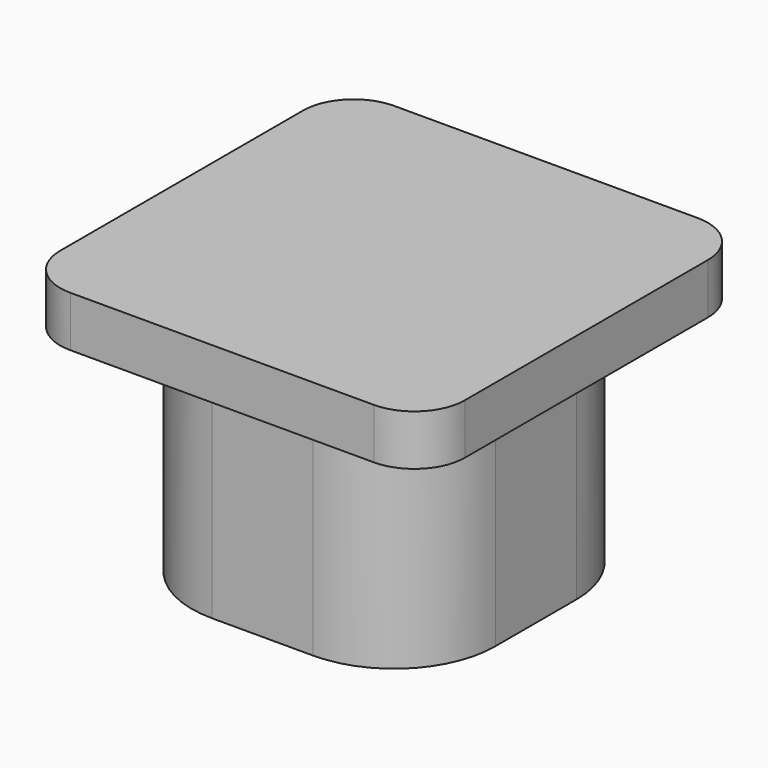
from build123d import *

# Parameters (mm, degrees)
F1_DEPTH     = 56.134
F3_DEPTH     = 12.7
F4_T         = 6.35
F4_T3_DEPTH  = 38.1
F4_T5_DEPTH  = 38.1
F4_T8_ANGLE  = 90.000000001
F4_T10_ANGLE = 90.000000001
F4_T12_ANGLE = 90.000000001
F4_T14_ANGLE = 90.000000001


# Not quite as in the source:
# - a shell that OpenCascade refuses in one call is made with other operations: the cavity is built on its own and cut out


with BuildPart() as f1:
    # F0 (on Top) → F1 (new body)
    with BuildSketch(Plane.XY):
        with BuildLine():
            ThreePointArc((-38.1, -12.7), (-30.6605122421, -30.6605122421), (-12.7, -38.1))
            Line((-12.7, -38.1), (12.7, -38.1))
            ThreePointArc((12.7, -38.1), (30.6605122421, -30.6605122421), (38.1, -12.7))
            Line((38.1, -12.7), (38.1, 12.7))
            ThreePointArc((38.1, 12.7), (30.6605122421, 30.6605122421), (12.7, 38.1))
            Line((12.7, 38.1), (-12.7, 38.1))
            ThreePointArc((-12.7, 38.1), (-30.6605122421, 30.6605122421), (-38.1, 12.7))
            Line((-38.1, 12.7), (-38.1, -12.7))
        make_face()
    extrude(amount=F1_DEPTH)

    # F2 (on face) → F3 (join)
    with BuildSketch(Plane.XY.offset(56.134)):
        with BuildLine():
            ThreePointArc((-50.8, -38.1), (-47.0802561211, -47.0802561211), (-38.1, -50.8))
            Line((-38.1, -50.8), (38.1, -50.8))
            ThreePointArc((38.1, -50.8), (47.0802561211, -47.0802561211), (50.8, -38.1))
            Line((50.8, -38.1), (50.8, 38.1))
            ThreePointArc((50.8, 38.1), (47.0802561211, 47.0802561211), (38.1, 50.8))
            Line((38.1, 50.8), (-38.1, 50.8))
            ThreePointArc((-38.1, 50.8), (-47.0802561211, 47.0802561211), (-50.8, 38.1))
            Line((-50.8, 38.1), (-50.8, -38.1))
        make_face()
    extrude(amount=F3_DEPTH)

    # F4: shell of thickness 6.35, made by hand


with BuildPart() as f4_core1:
    # F4_t2: copy of F1
    add(f1.part)

    # the walls: a layer under each face that stays
    f4_faces = [f4_core1.faces().sort_by_distance(p)[0] for p in [
        (-47.0802561211, -47.0802561211, 62.484),
        (-50.8, 0, 62.484),
        (0, -50.8, 62.484),
        (-33.8666666667, -33.8666666667, 56.134),
        (0, 0, 68.834),
        (-47.0802561211, 47.0802561211, 62.484),
        (47.0802561211, -47.0802561211, 62.484),
        (0, 50.8, 62.484),
        (50.8, 0, 62.484),
        (47.0802561211, 47.0802561211, 62.484),
        (-38.1, 0, 28.067),
        (-30.6605122421, -30.6605122421, 28.067),
        (0, -38.1, 28.067),
        (30.6605122421, -30.6605122421, 28.067),
        (38.1, 0, 28.067),
        (30.6605122421, 30.6605122421, 28.067),
        (0, 38.1, 28.067),
        (-30.6605122421, 30.6605122421, 28.067),
    ]]
    thicken(f4_faces, amount=-F4_T, mode=Mode.SUBTRACT)

    # F4_s4 → F4_t3 (cut)
    with BuildSketch(Plane.XZ.offset(-19.05)):
        Polygon((-38.1635, 56.0705), (-38.1, 62.484), (-31.75, 62.484), (-31.75, 56.134), align=None)
        Polygon((38.1635, 56.0705), (38.1, 62.484), (31.75, 62.484), (31.75, 56.134), align=None)
    extrude(amount=F4_T3_DEPTH, mode=Mode.SUBTRACT)

    # F4_s6 → F4_t5 (cut)
    with BuildSketch(Plane.YZ.offset(-19.05)):
        Polygon((-38.1635, 56.0705), (-38.1, 62.484), (-31.75, 62.484), (-31.75, 56.134), align=None)
        Polygon((38.1635, 56.0705), (38.1, 62.484), (31.75, 62.484), (31.75, 56.134), align=None)
    extrude(amount=F4_T5_DEPTH, mode=Mode.SUBTRACT)

    # F4_s7 → F4_t8 (revolve, cut)
    with BuildSketch(Plane.XZ.offset(12.7)):
        Polygon((-38.1635, 56.0705), (-38.1, 62.484), (-31.75, 62.484), (-31.75, 56.134), align=None)
    revolve(axis=Axis((-12.7, -12.7, 56.134), (0, 0, 1)), revolution_arc=F4_T8_ANGLE, mode=Mode.SUBTRACT)

    # F4_s9 → F4_t10 (revolve, cut)
    with BuildSketch(Plane.YZ.offset(12.7)):
        Polygon((-38.1635, 56.0705), (-38.1, 62.484), (-31.75, 62.484), (-31.75, 56.134), align=None)
    revolve(axis=Axis((12.7, -12.7, 56.134), (0, 0, 1)), revolution_arc=F4_T10_ANGLE, mode=Mode.SUBTRACT)

    # F4_s11 → F4_t12 (revolve, cut)
    with BuildSketch(Plane.XZ.offset(-12.7)):
        Polygon((38.1635, 56.0705), (38.1, 62.484), (31.75, 62.484), (31.75, 56.134), align=None)
    revolve(axis=Axis((12.7, 12.7, 56.134), (0, 0, 1)), revolution_arc=F4_T12_ANGLE, mode=Mode.SUBTRACT)

    # F4_s13 → F4_t14 (revolve, cut)
    with BuildSketch(Plane.YZ.offset(-12.7)):
        Polygon((38.1635, 56.0705), (38.1, 62.484), (31.75, 62.484), (31.75, 56.134), align=None)
    revolve(axis=Axis((-12.7, 12.7, 56.134), (0, 0, 1)), revolution_arc=F4_T14_ANGLE, mode=Mode.SUBTRACT)


with BuildPart() as f1_1:
    add(f1.part)

    # what is left inside the walls is the cavity
    f4_cavity = [f4_core1.part.solids().sort_by_distance(p)[0] for p in [
        (0, -10.583333, 62.4205),
    ]]
    add(f4_cavity, mode=Mode.SUBTRACT)


solid = f1_1.part
